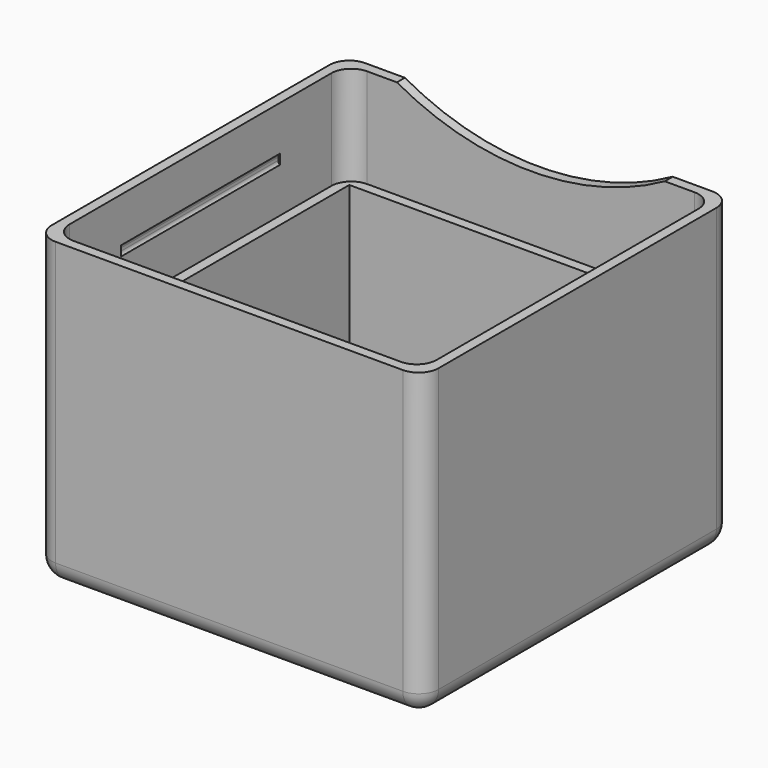
from build123d import *

# Parameters (mm, degrees)
F0_W         = 78
F0_H         = 78
F1_DEPTH     = 61
F2_T         = -4
F3_W         = 74
F3_H         = 74
F3_W_2       = 70
F3_H_2       = 70
F4_DEPTH     = 20
F6_DEPTH     = 2
F7_R         = 4
F8_R         = 4
F9_W         = 40
F9_H         = 2
F10_DEPTH    = 0.3
F11_T1_DEPTH = 43.5707142143


# Not quite as in the source:
# - a fillet or chamfer that OpenCascade refuses, or shapes differently, is made with other operations: its cross-section is extruded or revolved along the edge and cut away or added


with BuildPart() as f1:
    # F0 (on Top) → F1 (new body)
    with BuildSketch(Plane.XY):
        Rectangle(F0_W, F0_H)
    extrude(amount=F1_DEPTH)

    # F2
    f2_openings = [f1.faces().sort_by_distance(p)[0] for p in [
        (0, 0, 61),
    ]]
    offset(amount=F2_T, openings=f2_openings)

    # F3 (on face) → F4 (cut)
    with BuildSketch(Plane.XY.offset(61)):
        Rectangle(F3_W, F3_H)
        Rectangle(F3_W_2, F3_H_2, mode=Mode.SUBTRACT)
    extrude(amount=-F4_DEPTH, mode=Mode.SUBTRACT)

    # F5 (on face) → F6 (cut)
    with BuildSketch(Plane.XZ.offset(-37)):
        with BuildLine():
            Line((27, 61), (-27, 61))
            ThreePointArc((-27, 61), (0, 54), (27, 61))
        make_face()
    extrude(amount=-F6_DEPTH, mode=Mode.SUBTRACT)

    # F7
    f7_edges = [f1.edges().sort_by_distance(p)[0] for p in [
        (-39, 39, 30.5),
        (39, 39, 30.5),
        (39, -39, 30.5),
        (-39, -39, 30.5),
        (-39, 0, 0),
        (0, -39, 0),
        (39, 0, 0),
        (0, 39, 0),
    ]]
    fillet(f7_edges, radius=F7_R)

    # F8
    f8_edges = [f1.edges().sort_by_distance(p)[0] for p in [
        (37, -37, 51),
        (-37, -37, 51),
        (37, 37, 51),
        (-37, 37, 51),
    ]]
    fillet(f8_edges, radius=F8_R)

    # F9 (on face) → F10 (cut)
    with BuildSketch(Plane.YZ.offset(-37)):
        with Locations((0, 51)):
            Rectangle(F9_W, F9_H)
    extrude(amount=-F10_DEPTH, mode=Mode.SUBTRACT)

    # F11: fillet of radius 1 on 2 edges, made by hand

    # F11_s2 → F11_t1 (join)
    with BuildSketch(Plane.XZ.offset(-21.7853571071)):
        with BuildLine():
            ThreePointArc((-37, 50), (-37.2219544457, 50.3268445082), (-37.3, 50.7141428429))
            Line((-37.3, 50.7141428429), (-37.3, 50))
            Line((-37.3, 50), (-37, 50))
        make_face()
        with BuildLine():
            ThreePointArc((-37, 52), (-37.2219544457, 51.6731554918), (-37.3, 51.2858571571))
            Line((-37.3, 51.2858571571), (-37.3, 52))
            Line((-37.3, 52), (-37, 52))
        make_face()
    extrude(amount=F11_T1_DEPTH)


solid = f1.part
